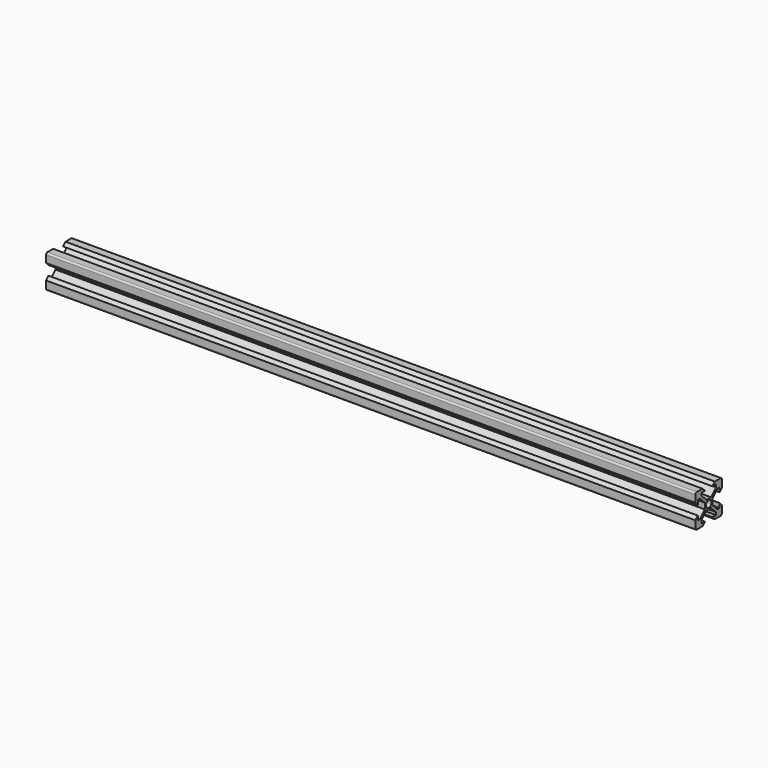
from build123d import *

# Parameters (mm, degrees)
F1_DEPTH = 391.8


# Not quite as in the source:
# - ends of sketch curves that miss each other by under 0.0002 mm in the source are joined


with BuildPart() as f1:
    # F0 (on Right) → F1 (new body)
    with BuildSketch(Plane.YZ):
        with BuildLine():
            Line((8.2, -10), (9, -10))
            ThreePointArc((9, -10), (9.7071067812, -9.7071067812), (10, -9))
            Line((10, -9), (10, -8.2))
            Line((10, -8.2), (8.2, -8.2))
            Line((8.2, -8.2), (8.2, -10))
        make_face()
        Polygon((5.4993398282, -8.2), (7.1393398282, -8.2), (5.4993398282, -6.56), align=None)
        Polygon((6.56, -5.4993398282), (8.2, -7.1393398282), (8.2, -5.4993398282), align=None)
        with BuildLine():
            Line((8.2, 10), (8.2, 8.2))
            Line((8.2, 8.2), (10, 8.2))
            Line((10, 8.2), (10, 9))
            ThreePointArc((10, 9), (9.7071067812, 9.7071067812), (9, 10))
            Line((9, 10), (8.2, 10))
        make_face()
        Polygon((8.2, 7.1393398282), (6.56, 5.4993398282), (8.2, 5.4993398282), align=None)
        Polygon((5.4993398282, 8.2), (5.4993398282, 6.56), (7.1393398282, 8.2), align=None)
        with BuildLine():
            Line((-9.9999004684, 8.2000055944), (-8.1999004684, 8.2000055944))
            Line((-8.1999004684, 8.2000055944), (-8.1999004684, 10.0000055944))
            Line((-8.1999004684, 10.0000055944), (-8.9999004684, 10.0000055944))
            ThreePointArc((-8.9999004684, 10.0000055944), (-9.7070072496, 9.7071123756), (-9.9999004684, 9.0000055944))
            Line((-9.9999004684, 9.0000055944), (-9.9999004684, 8.2000055944))
        make_face()
        Polygon((-7.1392402967, 8.2000055944), (-5.4992402967, 6.5600055944), (-5.4992402967, 8.2000055944), align=None)
        Polygon((-8.1999004684, 5.4993454226), (-6.5599004684, 5.4993454226), (-8.1999004684, 7.1393454226), align=None)
        with BuildLine():
            Line((-8.1999004684, -9.9999944056), (-8.1999004684, -8.1999944056))
            Line((-8.1999004684, -8.1999944056), (-9.9999004684, -8.1999944056))
            Line((-9.9999004684, -8.1999944056), (-9.9999004684, -8.9999944056))
            ThreePointArc((-9.9999004684, -8.9999944056), (-9.7070072496, -9.7071011868), (-8.9999004684, -9.9999944056))
            Line((-8.9999004684, -9.9999944056), (-8.1999004684, -9.9999944056))
        make_face()
        Polygon((-8.1999004684, -7.1393342338), (-6.5599004684, -5.4993342338), (-8.1999004684, -5.4993342338), align=None)
        Polygon((-5.4992402967, -8.1999944056), (-5.4992402967, -6.5599944056), (-7.1392402967, -8.1999944056), align=None)
        with BuildLine():
            Line((1.9173232366, -0.8566630648), (2.84, -1.7793398282))
            Line((2.84, -1.7793398282), (2.84, 0))
            Line((2.84, 0), (2.1, 0))
            ThreePointArc((2.1, 0), (2.0538231176, -0.4379618723), (1.9173232366, -0.8566630648))
        make_face()
        with BuildLine():
            Line((0, -2.84), (1.7793398282, -2.84))
            Line((1.7793398282, -2.84), (0.8566630648, -1.9173232366))
            ThreePointArc((0.8566630648, -1.9173232366), (0.4379618723, -2.0538231176), (0, -2.1))
            Line((0, -2.1), (0, -2.84))
        make_face()
        with BuildLine():
            Line((-1.7792402967, -2.8399944056), (9.95316e-05, -2.8399944056))
            Line((9.95316e-05, -2.8399944056), (0, -2.1))
            ThreePointArc((0, -2.1), (-0.4378623408, -2.0538175232), (-0.8565635332, -1.9173176422))
            Line((-0.8565635332, -1.9173176422), (-1.7792402967, -2.8399944056))
        make_face()
        Polygon((4.64, -10), (8.2, -10), (8.2, -8.2), (7.1393398282, -8.2), (5.4993398282, -8.2), (2.84, -8.2), align=None)
        Polygon((8.2, -8.2), (10, -8.2), (10, -4.64), (8.2, -2.84), (8.2, -5.4993398282), (8.2, -7.1393398282), align=None)
        with BuildLine():
            ThreePointArc((0, 2.1), (0.4379618723, 2.0538231176), (0.8566630648, 1.9173232366))
            Line((0.8566630648, 1.9173232366), (1.7793398282, 2.84))
            Line((1.7793398282, 2.84), (0, 2.84))
            Line((0, 2.84), (0, 2.1))
        make_face()
        with BuildLine():
            Line((2.1, 0), (2.84, 0))
            Line((2.84, 0), (2.84, 1.7793398282))
            Line((2.84, 1.7793398282), (1.9173232366, 0.8566630648))
            ThreePointArc((1.9173232366, 0.8566630648), (2.0538231176, 0.4379618723), (2.1, 0))
        make_face()
        with BuildLine():
            ThreePointArc((-0.8565635332, 1.917328831), (-0.4378623408, 2.053828712), (9.95316e-05, 2.1000055944))
            Line((9.95316e-05, 2.1000055944), (0, 2.84))
            Line((0, 2.84), (-1.7792402967, 2.8400055944))
            Line((-1.7792402967, 2.8400055944), (-0.8565635332, 1.917328831))
        make_face()
        Polygon((8.2, 8.2), (8.2, 7.1393398282), (8.2, 5.4993398282), (8.2, 2.84), (10, 4.64), (10, 8.2), align=None)
        Polygon((7.1393398282, 8.2), (8.2, 8.2), (8.2, 10), (4.64, 10), (2.84, 8.2), (5.4993398282, 8.2), align=None)
        with BuildLine():
            Line((-2.8399004684, 1.7793454226), (-2.8399004684, 5.5944e-06))
            Line((-2.8399004684, 5.5944e-06), (-2.0999004684, 5.5944e-06))
            ThreePointArc((-2.0999004684, 5.5944e-06), (-2.053723586, 0.4379674667), (-1.917223705, 0.8566686592))
            Line((-1.917223705, 0.8566686592), (-2.8399004684, 1.7793454226))
        make_face()
        Polygon((-8.1999004684, 10.0000055944), (-8.1999004684, 8.2000055944), (-7.1392402967, 8.2000055944), (-5.4992402967, 8.2000055944), (-2.8399004684, 8.2000055944), (-4.6399004684, 10.0000055944), align=None)
        Polygon((-8.1999004684, 5.4993454226), (-8.1999004684, 7.1393454226), (-8.1999004684, 8.2000055944), (-9.9999004684, 8.2000055944), (-9.9999004684, 4.6400055944), (-8.1999004684, 2.8400055944), align=None)
        with BuildLine():
            Line((-2.8399004684, 5.5944e-06), (-2.8399004684, -1.7793342338))
            Line((-2.8399004684, -1.7793342338), (-1.917223705, -0.8566574704))
            ThreePointArc((-1.917223705, -0.8566574704), (-2.053723586, -0.4379562779), (-2.0999004684, 5.5944e-06))
            Line((-2.0999004684, 5.5944e-06), (-2.8399004684, 5.5944e-06))
        make_face()
        Polygon((-9.9999004684, -8.1999944056), (-8.1999004684, -8.1999944056), (-8.1999004684, -7.1393342338), (-8.1999004684, -5.4993342338), (-8.1999004684, -2.8399944056), (-9.9999004684, -4.6399944056), align=None)
        Polygon((-5.4992402967, -8.1999944056), (-7.1392402967, -8.1999944056), (-8.1999004684, -8.1999944056), (-8.1999004684, -9.9999944056), (-4.6399004684, -9.9999944056), (-2.8399004684, -8.1999944056), align=None)
        with BuildLine():
            Line((-2.8399004684, -1.7793342338), (-1.7792402967, -2.8399944056))
            Line((-1.7792402967, -2.8399944056), (-0.8565635332, -1.9173176422))
            ThreePointArc((-0.8565635332, -1.9173176422), (-1.4848247089, -1.4849186461), (-1.917223705, -0.8566574704))
            Line((-1.917223705, -0.8566574704), (-2.8399004684, -1.7793342338))
        make_face()
        Polygon((-4.4695703825, -5.5303244915), (-1.7792402967, -2.8399944056), (-2.8399004684, -1.7793342338), (-5.5302305543, -4.4696643197), (-6.5599004684, -5.4993342338), (-8.1999004684, -7.1393342338), (-8.1999004684, -8.1999944056), (-7.1392402967, -8.1999944056), (-5.4992402967, -6.5599944056), align=None)
        with BuildLine():
            Line((7.1393398282, -8.2), (8.2, -8.2))
            Line((8.2, -8.2), (8.2, -7.1393398282))
            Line((8.2, -7.1393398282), (6.56, -5.4993398282))
            Line((6.56, -5.4993398282), (5.5303300859, -4.4696699141))
            Line((5.5303300859, -4.4696699141), (2.84, -1.7793398282))
            Line((2.84, -1.7793398282), (1.9173232366, -0.8566630648))
            ThreePointArc((1.9173232366, -0.8566630648), (1.4849242405, -1.4849242405), (0.8566630648, -1.9173232366))
            Line((0.8566630648, -1.9173232366), (1.7793398282, -2.84))
            Line((1.7793398282, -2.84), (4.4696699141, -5.5303300859))
            Line((4.4696699141, -5.5303300859), (5.4993398282, -6.56))
            Line((5.4993398282, -6.56), (7.1393398282, -8.2))
        make_face()
        with BuildLine():
            Line((1.9173232366, 0.8566630648), (2.84, 1.7793398282))
            Line((2.84, 1.7793398282), (5.5303300859, 4.4696699141))
            Line((5.5303300859, 4.4696699141), (6.56, 5.4993398282))
            Line((6.56, 5.4993398282), (8.2, 7.1393398282))
            Line((8.2, 7.1393398282), (8.2, 8.2))
            Line((8.2, 8.2), (7.1393398282, 8.2))
            Line((7.1393398282, 8.2), (5.4993398282, 6.56))
            Line((5.4993398282, 6.56), (4.4696699141, 5.5303300859))
            Line((4.4696699141, 5.5303300859), (1.7793398282, 2.84))
            Line((1.7793398282, 2.84), (0.8566630648, 1.9173232366))
            ThreePointArc((0.8566630648, 1.9173232366), (1.4849242405, 1.4849242405), (1.9173232366, 0.8566630648))
        make_face()
        with BuildLine():
            Line((-5.5302305543, 4.4696755085), (-2.8399004684, 1.7793454226))
            Line((-2.8399004684, 1.7793454226), (-1.917223705, 0.8566686592))
            ThreePointArc((-1.917223705, 0.8566686592), (-1.4848247089, 1.4849298349), (-0.8565635332, 1.917328831))
            Line((-0.8565635332, 1.917328831), (-1.7792402967, 2.8400055944))
            Line((-1.7792402967, 2.8400055944), (-4.4695703825, 5.5303356803))
            Line((-4.4695703825, 5.5303356803), (-5.4992402967, 6.5600055944))
            Line((-5.4992402967, 6.5600055944), (-7.1392402967, 8.2000055944))
            Line((-7.1392402967, 8.2000055944), (-8.1999004684, 8.2000055944))
            Line((-8.1999004684, 8.2000055944), (-8.1999004684, 7.1393454226))
            Line((-8.1999004684, 7.1393454226), (-6.5599004684, 5.4993454226))
            Line((-6.5599004684, 5.4993454226), (-5.5302305543, 4.4696755085))
        make_face()
    extrude(amount=F1_DEPTH)


solid = f1.part
